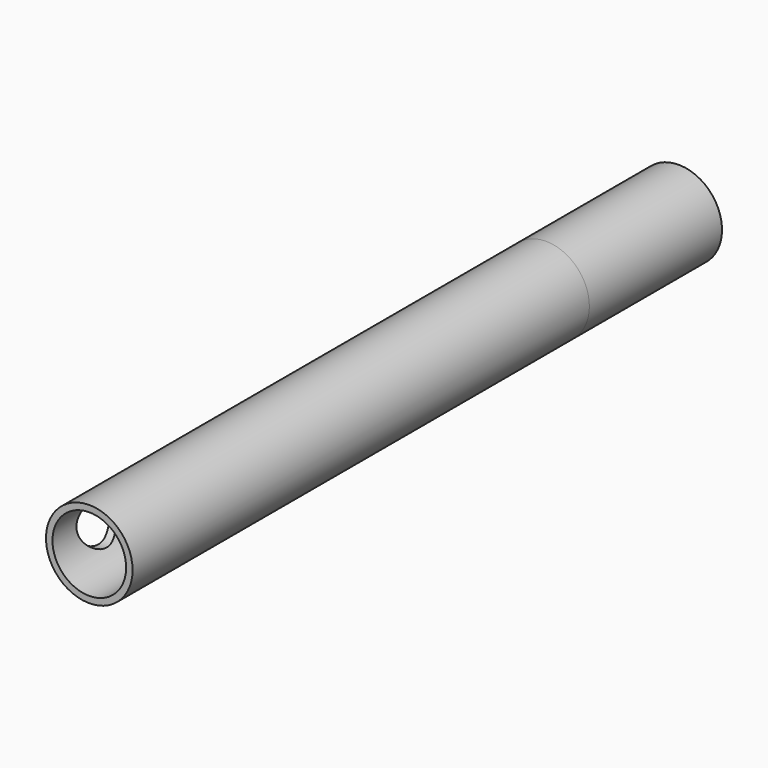
from build123d import *

# Parameters (mm, degrees)
F3_R      = 4.7
F4_DEPTH  = 37
F8_DEPTH  = 37
F6_R      = 4.7
F6_R_2    = 4
F9_DEPTH  = 25
F7_R      = 4.7
F7_R_2    = 4
F10_DEPTH = 18
F11_R     = 2.75
F12_DEPTH = 4.701


# Not quite as in the source:
# - ends of sketch curves that miss each other by under 0.0002 mm in the source are joined


with BuildPart() as f4:
    # F3 (on Front) → F4 (new body)
    with BuildSketch(Plane.XZ):
        Circle(F3_R)
    extrude(amount=F4_DEPTH)

    # F5 (on face) → F8 (cut, through all)
    with BuildSketch(Plane.XZ.offset(37)):
        with BuildLine():
            Line((-1.25, -3.8), (0, -3.8))
            Line((0, -3.8), (1.25, -3.8))
            Line((1.25, -3.8), (1.25, -3.7))
            ThreePointArc((1.25, -3.7), (1.3085786438, -3.5585786438), (1.45, -3.5))
            Line((1.45, -3.5), (2, -3.5))
            Line((2, -3.5), (2, -3.05))
            ThreePointArc((2, -3.05), (2.0585786438, -2.9085786438), (2.2, -2.85))
            Line((2.2, -2.85), (3.15, -2.85))
            Line((3.15, -2.85), (3.15, -2.15))
            Line((3.15, -2.15), (2.2, -2.15))
            ThreePointArc((2.2, -2.15), (2.0585786438, -2.0914213562), (2, -1.95))
            Line((2, -1.95), (2, -1.887459))
            ThreePointArc((2, -1.887459), (2.1033535752, -1.771554046), (2.2, -1.65))
            Line((2.2, -1.65), (3.75, -1.65))
            Line((3.75, -1.65), (3.75, 0))
            Line((3.75, 0), (3.75, 1.65))
            Line((3.75, 1.65), (2.2, 1.65))
            ThreePointArc((2.2, 1.65), (2.1033535752, 1.771554046), (1.9999998047, 1.8874588157))
            Line((1.9999998047, 1.8874588157), (2, 1.95))
            ThreePointArc((2, 1.95), (2.0585786438, 2.0914213562), (2.2, 2.15))
            Line((2.2, 2.15), (3.15, 2.15))
            Line((3.15, 2.15), (3.15, 2.85))
            Line((3.15, 2.85), (2.2, 2.85))
            ThreePointArc((2.2, 2.85), (2.0585786438, 2.9085786438), (2, 3.05))
            Line((2, 3.05), (2, 3.5))
            Line((2, 3.5), (1.45, 3.5))
            ThreePointArc((1.45, 3.5), (1.3085786438, 3.5585786438), (1.25, 3.7))
            Line((1.25, 3.7), (1.25, 3.8))
            Line((1.25, 3.8), (0, 3.8))
            Line((0, 3.8), (-1.25, 3.8))
            Line((-1.25, 3.8), (-1.25, 3.7))
            ThreePointArc((-1.25, 3.7), (-1.3085786438, 3.5585786438), (-1.45, 3.5))
            Line((-1.45, 3.5), (-2, 3.5))
            Line((-2, 3.5), (-2, 3.05))
            ThreePointArc((-2, 3.05), (-2.0585786438, 2.9085786438), (-2.2, 2.85))
            Line((-2.2, 2.85), (-3.15, 2.85))
            Line((-3.15, 2.85), (-3.15, 2.15))
            Line((-3.15, 2.15), (-2.2, 2.15))
            ThreePointArc((-2.2, 2.15), (-2.0585786438, 2.0914213562), (-2, 1.95))
            Line((-2, 1.95), (-2, 1.887459))
            ThreePointArc((-2, 1.887459), (-2.1033535752, 1.771554046), (-2.2, 1.65))
            Line((-2.2, 1.65), (-3.75, 1.65))
            Line((-3.75, 1.65), (-3.75, 0))
            Line((-3.75, 0), (-3.75, -1.65))
            Line((-3.75, -1.65), (-2.2, -1.65))
            ThreePointArc((-2.2, -1.65), (-2.1033535752, -1.771554046), (-1.9999998047, -1.8874588157))
            Line((-1.9999998047, -1.8874588157), (-2, -1.95))
            ThreePointArc((-2, -1.95), (-2.0585786438, -2.0914213562), (-2.2, -2.15))
            Line((-2.2, -2.15), (-3.15, -2.15))
            Line((-3.15, -2.15), (-3.15, -2.85))
            Line((-3.15, -2.85), (-2.2, -2.85))
            ThreePointArc((-2.2, -2.85), (-2.0585786438, -2.9085786438), (-2, -3.05))
            Line((-2, -3.05), (-2, -3.5))
            Line((-2, -3.5), (-1.45, -3.5))
            ThreePointArc((-1.45, -3.5), (-1.3085786438, -3.5585786438), (-1.25, -3.7))
            Line((-1.25, -3.7), (-1.25, -3.8))
        make_face()
    extrude(amount=-F8_DEPTH, mode=Mode.SUBTRACT)

    # F6 (on face) → F9 (join)
    with BuildSketch(Plane.XZ.offset(37)):
        Circle(F6_R)
        Circle(F6_R_2, mode=Mode.SUBTRACT)
    extrude(amount=F9_DEPTH)

    # F7 (on face) → F10 (join)
    with BuildSketch(Plane(origin=(0, 0, 0), x_dir=(-1, 0, 0), z_dir=(0, 1, 0))):
        Circle(F7_R)
        Circle(F7_R_2, mode=Mode.SUBTRACT)
    extrude(amount=F10_DEPTH)

    # F11 (on Right) → F12 (cut, through all)
    with BuildSketch(Plane.YZ):
        with Locations((-56, 0)):
            Circle(F11_R)
    extrude(amount=-F12_DEPTH, mode=Mode.SUBTRACT)


solid = f4.part
